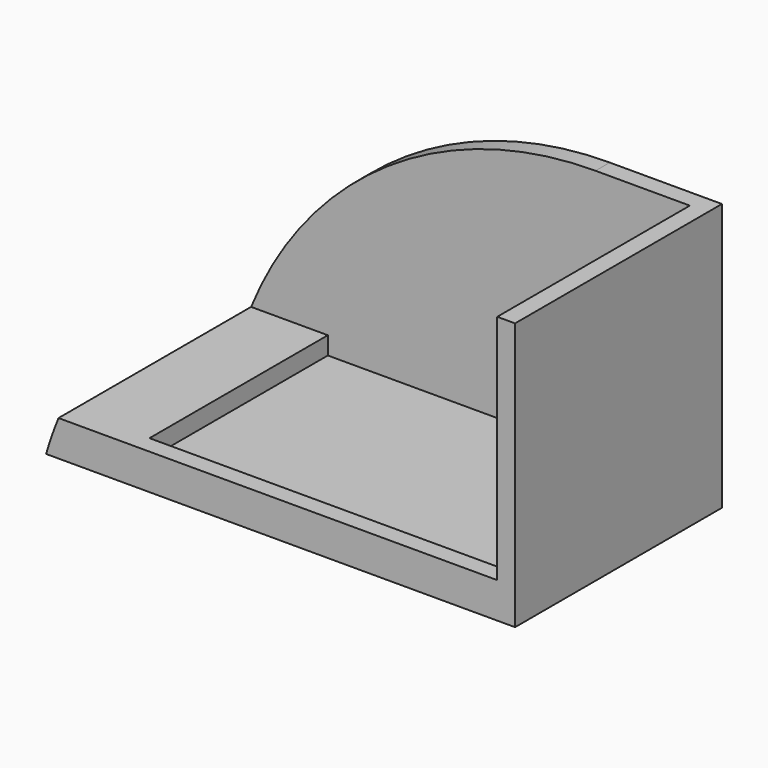
from build123d import *

# Parameters (mm, degrees)
F0_W        = 40.6
F0_H        = 25
F1_DEPTH    = 2
F2_DEPTH    = 30
F3_DEPTH    = 4
F4_DEPTH    = 30
F0_W_2      = 10
F5_DEPTH    = 4
F6_T1_DEPTH = 202.1185772835


# Not quite as in the source:
# - a fillet or chamfer that OpenCascade refuses, or shapes differently, is made with other operations: its cross-section is extruded or revolved along the edge and cut away or added


with BuildPart() as f1:
    # F0 (on Top) → F1 (new body)
    with BuildSketch(Plane.XY):
        with Locations((24.0341860496, -16.1564178318)):
            Rectangle(F0_W, F0_H)
    extrude(amount=F1_DEPTH)

    # F0 (on Top) → F2 (join)
    with BuildSketch(Plane.XY):
        Polygon((44.3341860496, -1.6564178318), (44.3341860496, -3.6564178318), (44.3341860496, -28.6564178318), (44.3341860496, -30.6564178318), (46.3341860496, -30.6564178318), (46.3341860496, -1.6564178318), align=None)
    extrude(amount=F2_DEPTH)

    # F0 (on Top) → F3 (join)
    with BuildSketch(Plane.XY):
        Polygon((44.3341860496, -28.6564178318), (3.7341860496, -28.6564178318), (-6.2658139504, -28.6564178318), (-6.2658139504, -30.6564178318), (44.3341860496, -30.6564178318), align=None)
    extrude(amount=F3_DEPTH)

    # F0 (on Top) → F4 (join)
    with BuildSketch(Plane.XY):
        Polygon((-6.2658139504, -3.6564178318), (3.7341860496, -3.6564178318), (44.3341860496, -3.6564178318), (44.3341860496, -1.6564178318), (-6.2658139504, -1.6564178318), align=None)
    extrude(amount=F4_DEPTH)

    # F0 (on Top) → F5 (join)
    with BuildSketch(Plane.XY):
        with Locations((-1.2658139504, -16.1564178318)):
            Rectangle(F0_W_2, F0_H)
    extrude(amount=F5_DEPTH)

    # F6: fillet of radius 41.6982966493 on 1 edges, made by hand

    # F6_s2 → F6_t1 (cut)
    with BuildSketch(Plane.XZ.offset(-98.40287081)):
        with BuildLine():
            ThreePointArc((-6.2658139504, 0), (8.7484143116, 21.6674566572), (33.7579015062, 30))
            Line((33.7579015062, 30), (-6.2658139504, 30))
            Line((-6.2658139504, 30), (-6.2658139504, 0))
        make_face()
    extrude(amount=F6_T1_DEPTH, mode=Mode.SUBTRACT)


solid = f1.part
